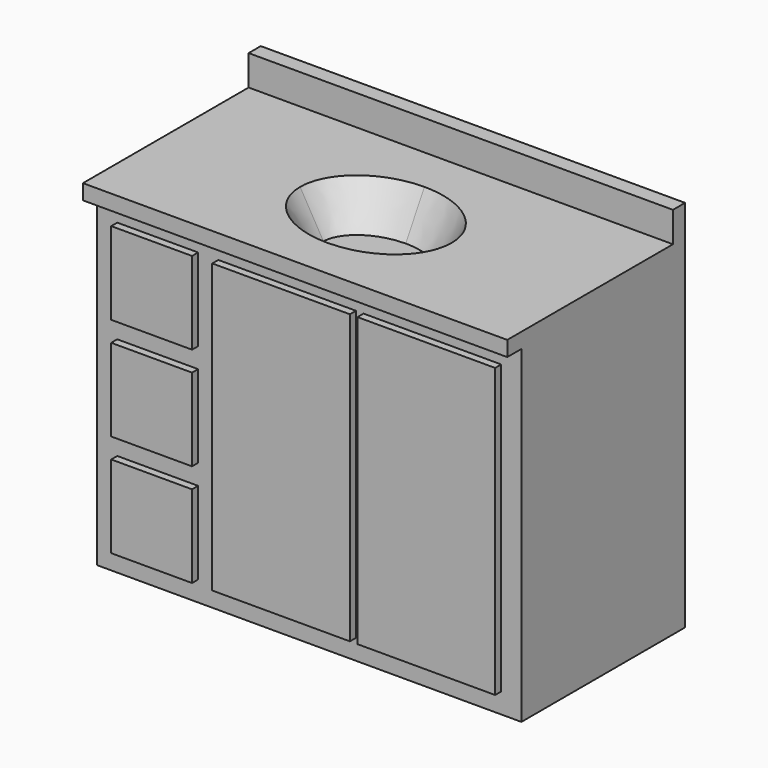
from build123d import *

# Parameters (mm, degrees)
F0_W     = 1066.8
F0_H     = 533.4
F1_DEPTH = 825.5
F2_W     = 1066.8
F2_H     = 558.8
F3_DEPTH = 38.1
F4_W     = 1066.8
F4_H     = 38.1
F5_DEPTH = 76.2
F6_W     = 1066.8
F6_H     = 825.5
F6_W_2   = 203.2
F6_H_2   = 207.4333333333
F6_W_3   = 346.075
F6_H_3   = 723.9
F7_DEPTH = 19.05
F9_DEPTH = 101.6
F9_TAPER = 30


with BuildPart() as f1:
    # F0 (on Top) → F1 (new body)
    with BuildSketch(Plane.XY):
        Rectangle(F0_W, F0_H)
    extrude(amount=F1_DEPTH)

    # F2 (on face) → F3 (join)
    with BuildSketch(Plane.XY.offset(825.5)):
        with Locations((0, -12.7)):
            Rectangle(F2_W, F2_H)
    extrude(amount=F3_DEPTH)

    # F4 (on face) → F5 (join)
    with BuildSketch(Plane.XY.offset(863.6)):
        with Locations((0, 247.65)):
            Rectangle(F4_W, F4_H)
    extrude(amount=F5_DEPTH)

    # F6 (on face) → F7 (cut)
    with BuildSketch(Plane.XZ.offset(266.7)):
        with Locations((0, 412.75)):
            Rectangle(F6_W, F6_H)
        with Locations((-381, 154.5166666667)):
            Rectangle(F6_W_2, F6_H_2, mode=Mode.SUBTRACT)
        with Locations((-381, 412.75)):
            Rectangle(F6_W_2, F6_H_2, mode=Mode.SUBTRACT)
        with Locations((-55.5625, 412.75)):
            Rectangle(F6_W_3, F6_H_3, mode=Mode.SUBTRACT)
        with Locations((-381, 670.9833333333)):
            Rectangle(F6_W_2, F6_H_2, mode=Mode.SUBTRACT)
        with Locations((309.5625, 412.75)):
            Rectangle(F6_W_3, F6_H_3, mode=Mode.SUBTRACT)
    extrude(amount=-F7_DEPTH, mode=Mode.SUBTRACT)

    # F8 (on face) → F9 (cut)
    with BuildSketch(Plane.XY.offset(863.6)):
        with BuildLine():
            add(Edge.make_bspline(
                [(190.5, -38.1), (190.5, 225.8645430735), (-95.25, 93.8822715367), (-381, -38.1), (-95.25, -170.0822715367), (190.5, -302.0645430735), (190.5, -38.1)],
                knots=[0, 0, 0, 2.0943951024, 2.0943951024, 4.1887902048, 4.1887902048, 6.2831853072, 6.2831853072, 6.2831853072], degree=2, weights=[1, 0.5, 1, 0.5, 1, 0.5, 1]))
        make_face()
    extrude(amount=-F9_DEPTH, taper=F9_TAPER, mode=Mode.SUBTRACT)


solid = f1.part
